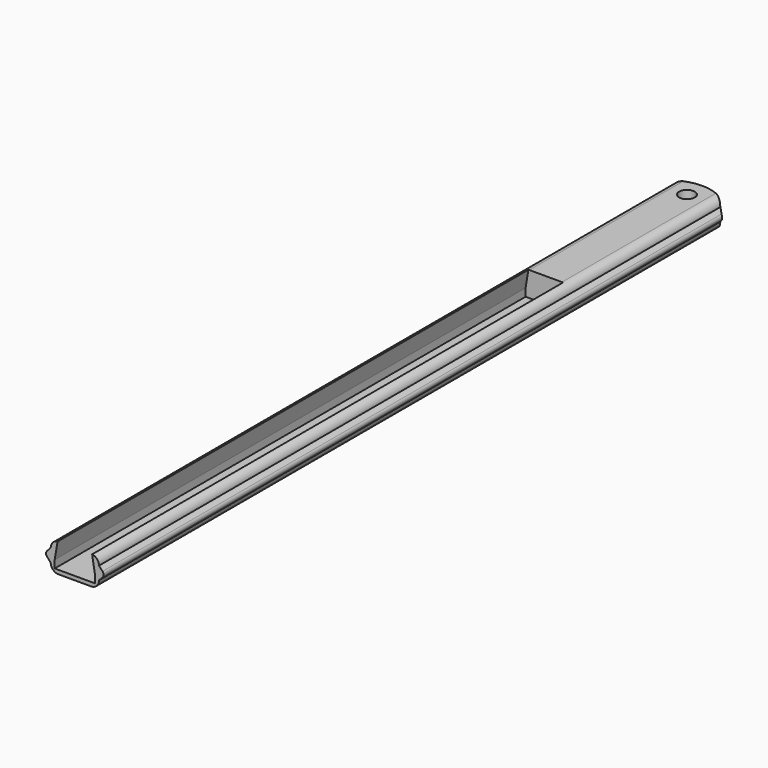
from build123d import *

# Parameters (mm, degrees)
F1_DEPTH = 200
F2_R     = 2
F3_DEPTH = 7.301
F6_DEPTH = 25
F9_DEPTH = 150


# Not quite as in the source:
# - a feature names something its author has since deleted; it is built from what else it names


with BuildPart() as f1:
    # F0 (on Front) → F1 (new body)
    with BuildSketch(Plane.XZ):
        with BuildLine():
            Line((7.0581561667, 0.685534298), (6.15, 1.65))
            ThreePointArc((6.15, 1.65), (5.5642135624, 3.0642135624), (4.15, 3.65))
            Line((4.15, 3.65), (-4.15, 3.65))
            ThreePointArc((-4.15, 3.65), (-5.5642135624, 3.0642135624), (-6.15, 1.65))
            Line((-6.15, 1.65), (-7.0581561667, 0.685534298))
            ThreePointArc((-7.0581561667, 0.685534298), (-7.3301158338, 0), (-7.0581561667, -0.685534298))
            Line((-7.0581561667, -0.685534298), (-6.15, -1.65))
            ThreePointArc((-6.15, -1.65), (-5.5642135624, -3.0642135624), (-4.15, -3.65))
            Line((-4.15, -3.65), (4.15, -3.65))
            ThreePointArc((4.15, -3.65), (5.5642135624, -3.0642135624), (6.15, -1.65))
            Line((6.15, -1.65), (7.0581561667, -0.685534298))
            ThreePointArc((7.0581561667, -0.685534298), (7.3301158338, 0), (7.0581561667, 0.685534298))
        make_face()
        with BuildLine():
            ThreePointArc((5.15, -1.65), (4.8571067812, -2.3571067812), (4.15, -2.65))
            Line((4.15, -2.65), (-4.15, -2.65))
            ThreePointArc((-4.15, -2.65), (-4.8571067812, -2.3571067812), (-5.15, -1.65))
            Line((-5.15, -1.65), (-5.15, 1.65))
            ThreePointArc((-5.15, 1.65), (-4.8571067812, 2.3571067812), (-4.15, 2.65))
            Line((-4.15, 2.65), (4.15, 2.65))
            ThreePointArc((4.15, 2.65), (4.8571067812, 2.3571067812), (5.15, 1.65))
            Line((5.15, 1.65), (5.15, -1.65))
        make_face(mode=Mode.SUBTRACT)
        with BuildLine():
            Line((-4.15, -2.65), (4.15, -2.65))
            ThreePointArc((4.15, -2.65), (4.8571067812, -2.3571067812), (5.15, -1.65))
            Line((5.15, -1.65), (5.15, 1.65))
            ThreePointArc((5.15, 1.65), (4.8571067812, 2.3571067812), (4.15, 2.65))
            Line((4.15, 2.65), (-4.15, 2.65))
            ThreePointArc((-4.15, 2.65), (-4.8571067812, 2.3571067812), (-5.15, 1.65))
            Line((-5.15, 1.65), (-5.15, -1.65))
            ThreePointArc((-5.15, -1.65), (-4.8571067812, -2.3571067812), (-4.15, -2.65))
        make_face()
    extrude(amount=F1_DEPTH)

    # F2 (on face) → F3 (cut, through all)
    with BuildSketch(Plane.XY.offset(3.65)):
        with Locations((0, -5)):
            Circle(F2_R)
    extrude(amount=-F3_DEPTH, mode=Mode.SUBTRACT)

    # F5 (on offset) → F6 (cut)
    with BuildSketch(Plane.XY.offset(4.6)):
        with BuildLine():
            Line((8, -3.7011680724), (8, 3.7011680724))
            Line((8, 3.7011680724), (-8, 3.7011680724))
            Line((-8, 3.7011680724), (-8, -3.7011680724))
            ThreePointArc((-8, -3.7011680724), (0, -0.1482238292), (8, -3.7011680724))
        make_face()
    extrude(amount=-F6_DEPTH, mode=Mode.SUBTRACT)

    # F8 (on offset) → F9 (cut)
    with BuildSketch(Plane.XZ.offset(200)):
        Polygon((-5.1262229681, -2.646596171), (0, -2.646596171), (5.1262229681, -2.646596171), (5.1262229681, -0.6600963534), (4.3867812492, 3.7468392402), (0, 3.7468392402), (-4.3867812492, 3.7468392402), (-5.1262229681, -0.6600963534), align=None)
    extrude(amount=-F9_DEPTH, mode=Mode.SUBTRACT)


solid = f1.part
